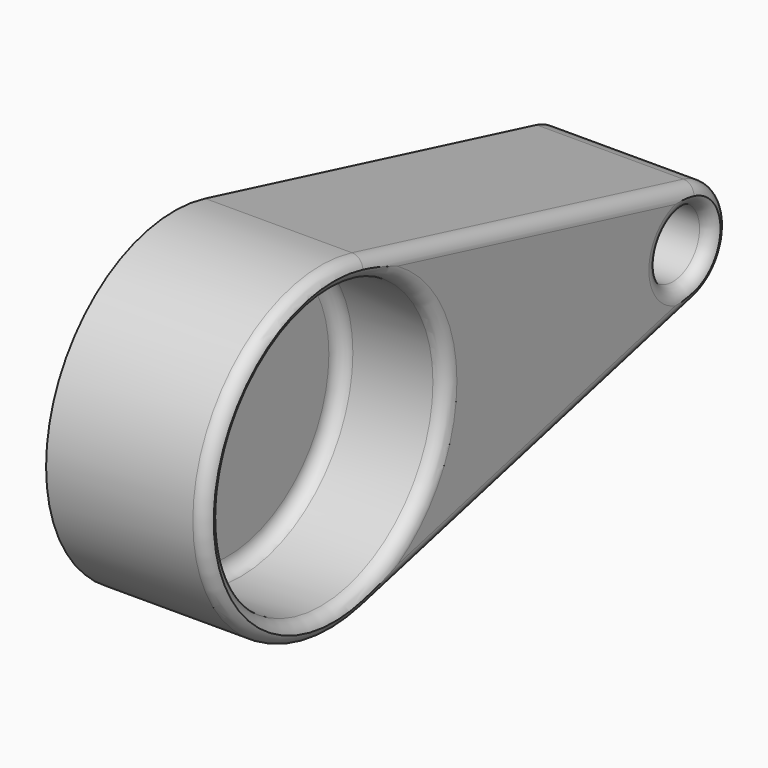
from build123d import *

# Parameters (mm, degrees)
F1_DEPTH = 76.2
F2_R     = 66.675
F2_R_2   = 15.875
F3_DEPTH = 50.8
F4_F1_R  = 6.35
F4_F2_R  = 6.35
F4_F3_R  = 6.35


# Not quite as in the source:
# - a fillet or chamfer that OpenCascade refuses, or shapes differently, is made with other operations: its cross-section is extruded or revolved along the edge and cut away or added


with BuildPart() as f1:
    # F0 (on Right) → F1 (new body)
    with BuildSketch(Plane.YZ):
        with BuildLine():
            ThreePointArc((18.4812146278, -73.9248585111), (60.0612543768, -46.8944103565), (76.2, 0))
            ThreePointArc((76.2, 0), (60.0612543768, 46.8944103565), (18.4812146278, 73.9248585111))
            ThreePointArc((18.4812146278, 73.9248585111), (-76.2, 0), (18.4812146278, -73.9248585111))
        make_face()
        with BuildLine():
            ThreePointArc((18.4812146278, 73.9248585111), (60.0612543768, 46.8944103565), (76.2, 0))
            ThreePointArc((76.2, 0), (60.0612543768, -46.8944103565), (18.4812146278, -73.9248585111))
            Line((18.4812146278, -73.9248585111), (215.6141706573, -24.6416195037))
            ThreePointArc((215.6141706573, -24.6416195037), (184.0537657814, 0), (215.6141706573, 24.6416195037))
            Line((215.6141706573, 24.6416195037), (18.4812146278, 73.9248585111))
        make_face()
        with BuildLine():
            ThreePointArc((234.8537657814, 0), (229.474183907, 15.6314701188), (215.6141706573, 24.6416195037))
            ThreePointArc((215.6141706573, 24.6416195037), (184.0537657814, 0), (215.6141706573, -24.6416195037))
            ThreePointArc((215.6141706573, -24.6416195037), (229.474183907, -15.6314701188), (234.8537657814, 0))
        make_face()
    extrude(amount=F1_DEPTH)

    # F2 (on face) → F3 (cut)
    with BuildSketch(Plane.YZ.offset(76.2)):
        Circle(F2_R)
        with Locations((209.4537657814, 0)):
            Circle(F2_R_2)
    extrude(amount=-F3_DEPTH, mode=Mode.SUBTRACT)

    # F4: fillet of radius 6.35 on 8 edges, made by hand

    # F4_f1
    f4_f1_edges = [f1.edges().sort_by_distance(p)[0] for p in [
        (76.2, -76.2, 0),
        (76.2, 117.0476926425, 49.2832390074),
        (76.2, 117.0476926425, -49.2832390074),
        (76.2, 234.8537657814, 0),
    ]]
    fillet(f4_f1_edges, radius=F4_F1_R)

    # F4_f2
    f4_f2_edges = [f1.edges().sort_by_distance(p)[0] for p in [
        (25.4, -66.675, 0),
    ]]
    fillet(f4_f2_edges, radius=F4_F2_R)

    # F4_f3
    f4_f3_edges = [f1.edges().sort_by_distance(p)[0] for p in [
        (25.4, 193.5787657814, 0),
    ]]
    fillet(f4_f3_edges, radius=F4_F3_R)

    # F4_s4 → F4_t5 (revolve, cut)
    with BuildSketch(Plane.XY):
        with BuildLine():
            ThreePointArc((76.2, 73.025), (74.3401280605, 68.5348719395), (69.85, 66.675))
            Line((69.85, 66.675), (69.85, 66.548))
            Line((69.85, 66.548), (76.327, 66.548))
            Line((76.327, 66.548), (76.327, 73.025))
            Line((76.327, 73.025), (76.2, 73.025))
        make_face()
    revolve(axis=Axis((76.2, 0, 0), (1, 0, 0)), mode=Mode.SUBTRACT)

    # F4_s6 → F4_t7 (revolve, cut)
    with BuildSketch(Plane.XY):
        with BuildLine():
            ThreePointArc((69.85, 225.3287657814), (74.3401280605, 227.1886377208), (76.2, 231.6787657814))
            Line((76.2, 231.6787657814), (76.327, 231.6787657814))
            Line((76.327, 231.6787657814), (76.327, 225.2017657814))
            Line((76.327, 225.2017657814), (69.85, 225.2017657814))
            Line((69.85, 225.2017657814), (69.85, 225.3287657814))
        make_face()
    revolve(axis=Axis((76.2, 209.4537657814, 0), (1, 0, 0)), mode=Mode.SUBTRACT)


solid = f1.part
